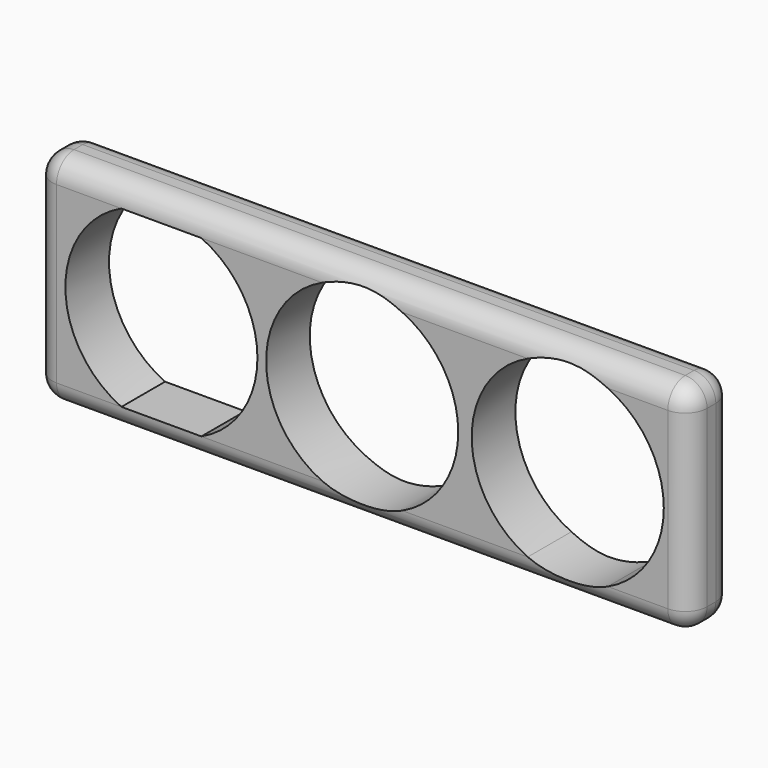
from build123d import *

# Parameters (mm, degrees)
F0_W         = 76.2
F0_H         = 25.4
F0_R         = 11.176
F1_DEPTH     = 6.35
F2_T1_DEPTH  = 71.12
F2_T3_DEPTH  = 1.27
F2_T5_DEPTH  = 20.32
F2_S9_W      = 2.54
F2_S9_H      = 2.54
F2_T10_DEPTH = 2.54
F2_S15_W     = 2.54
F2_S15_H     = 2.54
F2_T16_DEPTH = 2.54
F2_S21_W     = 2.54
F2_S21_H     = 2.54
F2_T22_DEPTH = 2.54
F2_S27_W     = 2.54
F2_S27_H     = 2.54
F2_T28_DEPTH = 2.54
F2_S33_W     = 2.54
F2_S33_H     = 2.54
F2_T34_DEPTH = 2.54
F2_S39_W     = 2.54
F2_S39_H     = 2.54
F2_T40_DEPTH = 2.54
F2_S45_W     = 2.54
F2_S45_H     = 2.54
F2_T46_DEPTH = 2.54
F2_S51_W     = 2.54
F2_S51_H     = 2.54
F2_T52_DEPTH = 2.54
F4_DEPTH     = 6.35


# Not quite as in the source:
# - a fillet or chamfer that OpenCascade refuses, or shapes differently, is made with other operations: its cross-section is extruded or revolved along the edge and cut away or added


with BuildPart() as f1:
    # F0 (on Front) → F1 (new body)
    with BuildSketch(Plane.XZ):
        Rectangle(F0_W, F0_H)
        Circle(F0_R, mode=Mode.SUBTRACT)
    extrude(amount=F1_DEPTH)

    # F2: fillet of radius 2.54 on 12 edges, made by hand

    # F2_s2 → F2_t1 (cut)
    with BuildSketch(Plane.YZ.offset(-35.56)):
        with BuildLine():
            ThreePointArc((-2.54, -12.7), (-0.7439487758, -11.9560512242), (0, -10.16))
            Line((0, -10.16), (0, -12.7))
            Line((0, -12.7), (-2.54, -12.7))
        make_face()
        with BuildLine():
            ThreePointArc((-3.81, -12.7), (-5.6060512242, -11.9560512242), (-6.35, -10.16))
            Line((-6.35, -10.16), (-6.35, -12.7))
            Line((-6.35, -12.7), (-3.81, -12.7))
        make_face()
        with BuildLine():
            ThreePointArc((-2.54, 12.7), (-0.7439487758, 11.9560512242), (0, 10.16))
            Line((0, 10.16), (0, 12.7))
            Line((0, 12.7), (-2.54, 12.7))
        make_face()
        with BuildLine():
            ThreePointArc((-3.81, 12.7), (-5.6060512242, 11.9560512242), (-6.35, 10.16))
            Line((-6.35, 10.16), (-6.35, 12.7))
            Line((-6.35, 12.7), (-3.81, 12.7))
        make_face()
    extrude(amount=F2_T1_DEPTH, mode=Mode.SUBTRACT)

    # F2_s4 → F2_t3 (cut)
    with BuildSketch(Plane.XZ.offset(2.54)):
        with BuildLine():
            ThreePointArc((-38.1, -10.16), (-37.3560512242, -11.9560512242), (-35.56, -12.7))
            Line((-35.56, -12.7), (-38.1, -12.7))
            Line((-38.1, -12.7), (-38.1, -10.16))
        make_face()
        with BuildLine():
            ThreePointArc((38.1, -10.16), (37.3560512242, -11.9560512242), (35.56, -12.7))
            Line((35.56, -12.7), (38.1, -12.7))
            Line((38.1, -12.7), (38.1, -10.16))
        make_face()
        with BuildLine():
            ThreePointArc((38.1, 10.16), (37.3560512242, 11.9560512242), (35.56, 12.7))
            Line((35.56, 12.7), (38.1, 12.7))
            Line((38.1, 12.7), (38.1, 10.16))
        make_face()
        with BuildLine():
            ThreePointArc((-35.56, 12.7), (-37.3560512242, 11.9560512242), (-38.1, 10.16))
            Line((-38.1, 10.16), (-38.1, 12.7))
            Line((-38.1, 12.7), (-35.56, 12.7))
        make_face()
    extrude(amount=F2_T3_DEPTH, mode=Mode.SUBTRACT)

    # F2_s6 → F2_t5 (cut)
    with BuildSketch(Plane.XY.offset(-10.16)):
        with BuildLine():
            ThreePointArc((-38.1, -3.81), (-37.3560512242, -5.6060512242), (-35.56, -6.35))
            Line((-35.56, -6.35), (-38.1, -6.35))
            Line((-38.1, -6.35), (-38.1, -3.81))
        make_face()
        with BuildLine():
            ThreePointArc((-38.1, -2.54), (-37.3560512242, -0.7439487758), (-35.56, 0))
            Line((-35.56, 0), (-38.1, 0))
            Line((-38.1, 0), (-38.1, -2.54))
        make_face()
        with BuildLine():
            ThreePointArc((38.1, -3.81), (37.3560512242, -5.6060512242), (35.56, -6.35))
            Line((35.56, -6.35), (38.1, -6.35))
            Line((38.1, -6.35), (38.1, -3.81))
        make_face()
        with BuildLine():
            ThreePointArc((38.1, -2.54), (37.3560512242, -0.7439487758), (35.56, 0))
            Line((35.56, 0), (38.1, 0))
            Line((38.1, 0), (38.1, -2.54))
        make_face()
    extrude(amount=F2_T5_DEPTH, mode=Mode.SUBTRACT)


with BuildPart() as f2_tool8:
    # F2_s9 → F2_t10 (new body)
    with BuildSketch(Plane.YZ.offset(-35.56)):
        with Locations((-1.27, -11.43)):
            Rectangle(F2_S9_W, F2_S9_H)
    extrude(amount=-F2_T10_DEPTH)

    # F2_s11 → F2_t12 (revolve, cut)
    with BuildSketch(Plane(origin=(-35.56, -2.54, -10.16), x_dir=(0, -0.7071067812, 0.7071067812), z_dir=(0, -0.7071067812, -0.7071067812))):
        with BuildLine():
            ThreePointArc((0, -2.54), (2.54, 0), (0, 2.54))
            Line((0, 2.54), (0, -2.54))
        make_face()
    revolve(axis=Axis((-35.56, -2.54, -10.16), (-1, 0, 0)), mode=Mode.SUBTRACT)


with BuildPart() as f1_1:
    add(f1.part)

    # F2_t7: cut F2_tool8
    add(f2_tool8.part, mode=Mode.SUBTRACT)


with BuildPart() as f2_tool14:
    # F2_s15 → F2_t16 (new body)
    with BuildSketch(Plane.YZ.offset(35.56)):
        with Locations((-1.27, -11.43)):
            Rectangle(F2_S15_W, F2_S15_H)
    extrude(amount=F2_T16_DEPTH)

    # F2_s17 → F2_t18 (revolve, cut)
    with BuildSketch(Plane(origin=(35.56, -2.54, -10.16), x_dir=(0, -0.7071067812, 0.7071067812), z_dir=(0, 0.7071067812, 0.7071067812))):
        with BuildLine():
            ThreePointArc((0, -2.54), (2.54, 0), (0, 2.54))
            Line((0, 2.54), (0, -2.54))
        make_face()
    revolve(axis=Axis((35.56, -2.54, -10.16), (1, 0, 0)), mode=Mode.SUBTRACT)


with BuildPart() as f1_2:
    add(f1_1.part)

    # F2_t13: cut F2_tool14
    add(f2_tool14.part, mode=Mode.SUBTRACT)


with BuildPart() as f2_tool20:
    # F2_s21 → F2_t22 (new body)
    with BuildSketch(Plane.YZ.offset(-35.56)):
        with Locations((-5.08, -11.43)):
            Rectangle(F2_S21_W, F2_S21_H)
    extrude(amount=-F2_T22_DEPTH)

    # F2_s23 → F2_t24 (revolve, cut)
    with BuildSketch(Plane(origin=(-35.56, -3.81, -10.16), x_dir=(0, 0.7071067812, 0.7071067812), z_dir=(0, -0.7071067812, 0.7071067812))):
        with BuildLine():
            ThreePointArc((0, -2.54), (2.54, 0), (0, 2.54))
            Line((0, 2.54), (0, -2.54))
        make_face()
    revolve(axis=Axis((-35.56, -3.81, -10.16), (-1, 0, 0)), mode=Mode.SUBTRACT)


with BuildPart() as f1_3:
    add(f1_2.part)

    # F2_t19: cut F2_tool20
    add(f2_tool20.part, mode=Mode.SUBTRACT)


with BuildPart() as f2_tool26:
    # F2_s27 → F2_t28 (new body)
    with BuildSketch(Plane.YZ.offset(35.56)):
        with Locations((-5.08, -11.43)):
            Rectangle(F2_S27_W, F2_S27_H)
    extrude(amount=F2_T28_DEPTH)

    # F2_s29 → F2_t30 (revolve, cut)
    with BuildSketch(Plane(origin=(35.56, -3.81, -10.16), x_dir=(0, 0.7071067812, 0.7071067812), z_dir=(0, 0.7071067812, -0.7071067812))):
        with BuildLine():
            ThreePointArc((0, -2.54), (2.54, 0), (0, 2.54))
            Line((0, 2.54), (0, -2.54))
        make_face()
    revolve(axis=Axis((35.56, -3.81, -10.16), (1, 0, 0)), mode=Mode.SUBTRACT)


with BuildPart() as f1_4:
    add(f1_3.part)

    # F2_t25: cut F2_tool26
    add(f2_tool26.part, mode=Mode.SUBTRACT)


with BuildPart() as f2_tool32:
    # F2_s33 → F2_t34 (new body)
    with BuildSketch(Plane.XY.offset(10.16)):
        with Locations((-36.83, -5.08)):
            Rectangle(F2_S33_W, F2_S33_H)
    extrude(amount=F2_T34_DEPTH)

    # F2_s35 → F2_t36 (revolve, cut)
    with BuildSketch(Plane(origin=(-35.56, -3.81, 10.16), x_dir=(0.7071067812, 0.7071067812, 0), z_dir=(0.7071067812, -0.7071067812, 0))):
        with BuildLine():
            ThreePointArc((0, -2.54), (2.54, 0), (0, 2.54))
            Line((0, 2.54), (0, -2.54))
        make_face()
    revolve(axis=Axis((-35.56, -3.81, 10.16), (0, 0, 1)), mode=Mode.SUBTRACT)


with BuildPart() as f1_5:
    add(f1_4.part)

    # F2_t31: cut F2_tool32
    add(f2_tool32.part, mode=Mode.SUBTRACT)


with BuildPart() as f2_tool38:
    # F2_s39 → F2_t40 (new body)
    with BuildSketch(Plane.XY.offset(10.16)):
        with Locations((-36.83, -1.27)):
            Rectangle(F2_S39_W, F2_S39_H)
    extrude(amount=F2_T40_DEPTH)

    # F2_s41 → F2_t42 (revolve, cut)
    with BuildSketch(Plane(origin=(-35.56, -2.54, 10.16), x_dir=(0.7071067812, -0.7071067812, 0), z_dir=(-0.7071067812, -0.7071067812, 0))):
        with BuildLine():
            ThreePointArc((0, -2.54), (2.54, 0), (0, 2.54))
            Line((0, 2.54), (0, -2.54))
        make_face()
    revolve(axis=Axis((-35.56, -2.54, 10.16), (0, 0, 1)), mode=Mode.SUBTRACT)


with BuildPart() as f1_6:
    add(f1_5.part)

    # F2_t37: cut F2_tool38
    add(f2_tool38.part, mode=Mode.SUBTRACT)


with BuildPart() as f2_tool44:
    # F2_s45 → F2_t46 (new body)
    with BuildSketch(Plane.YZ.offset(35.56)):
        with Locations((-5.08, 11.43)):
            Rectangle(F2_S45_W, F2_S45_H)
    extrude(amount=F2_T46_DEPTH)

    # F2_s47 → F2_t48 (revolve, cut)
    with BuildSketch(Plane(origin=(35.56, -3.81, 10.16), x_dir=(0, 0.7071067812, -0.7071067812), z_dir=(0, -0.7071067812, -0.7071067812))):
        with BuildLine():
            ThreePointArc((0, -2.54), (2.54, 0), (0, 2.54))
            Line((0, 2.54), (0, -2.54))
        make_face()
    revolve(axis=Axis((35.56, -3.81, 10.16), (1, 0, 0)), mode=Mode.SUBTRACT)


with BuildPart() as f1_7:
    add(f1_6.part)

    # F2_t43: cut F2_tool44
    add(f2_tool44.part, mode=Mode.SUBTRACT)


with BuildPart() as f2_tool50:
    # F2_s51 → F2_t52 (new body)
    with BuildSketch(Plane.YZ.offset(35.56)):
        with Locations((-1.27, 11.43)):
            Rectangle(F2_S51_W, F2_S51_H)
    extrude(amount=F2_T52_DEPTH)

    # F2_s53 → F2_t54 (revolve, cut)
    with BuildSketch(Plane(origin=(35.56, -2.54, 10.16), x_dir=(0, -0.7071067812, -0.7071067812), z_dir=(0, -0.7071067812, 0.7071067812))):
        with BuildLine():
            ThreePointArc((0, -2.54), (2.54, 0), (0, 2.54))
            Line((0, 2.54), (0, -2.54))
        make_face()
    revolve(axis=Axis((35.56, -2.54, 10.16), (1, 0, 0)), mode=Mode.SUBTRACT)


with BuildPart() as f1_8:
    add(f1_7.part)

    # F2_t49: cut F2_tool50
    add(f2_tool50.part, mode=Mode.SUBTRACT)

    # F3 (on face) → F4 (cut)
    with BuildSketch(Plane.XZ.offset(6.35)):
        with BuildLine():
            ThreePointArc((-18.7094612276, -10.16), (-13.9572398788, -6.0369996274), (-12.1859761156, 0))
            ThreePointArc((-12.1859761156, 0), (-13.9572398788, 6.0369996274), (-18.7094612276, 10.16))
            Line((-18.7094612276, 10.16), (-28.0096651758, 10.16))
            ThreePointArc((-28.0096651758, 10.16), (-34.5331502877, 0), (-28.0096651758, -10.16))
            Line((-28.0096651758, -10.16), (-18.7094612276, -10.16))
        make_face()
        with BuildLine():
            ThreePointArc((28.5749689082, -10.16), (33.3248489457, -6.0360861565), (35.0950720022, 0))
            ThreePointArc((35.0950720022, 0), (33.3248489457, 6.0360861565), (28.5749689082, 10.16))
            Line((28.5749689082, 10.16), (19.2631750961, 10.16))
            ThreePointArc((19.2631750961, 10.16), (12.7430720022, 0), (19.2631750961, -10.16))
            Line((19.2631750961, -10.16), (28.5749689082, -10.16))
        make_face()
        with BuildLine():
            Line((19.2631750961, 10.16), (28.5749689082, 10.16))
            ThreePointArc((28.5749689082, 10.16), (23.9190720022, 11.176), (19.2631750961, 10.16))
        make_face()
        with BuildLine():
            ThreePointArc((19.2631750961, -10.16), (23.9190720022, -11.176), (28.5749689082, -10.16))
            Line((28.5749689082, -10.16), (19.2631750961, -10.16))
        make_face()
    extrude(amount=-F4_DEPTH, mode=Mode.SUBTRACT)


solid = f1_8.part
